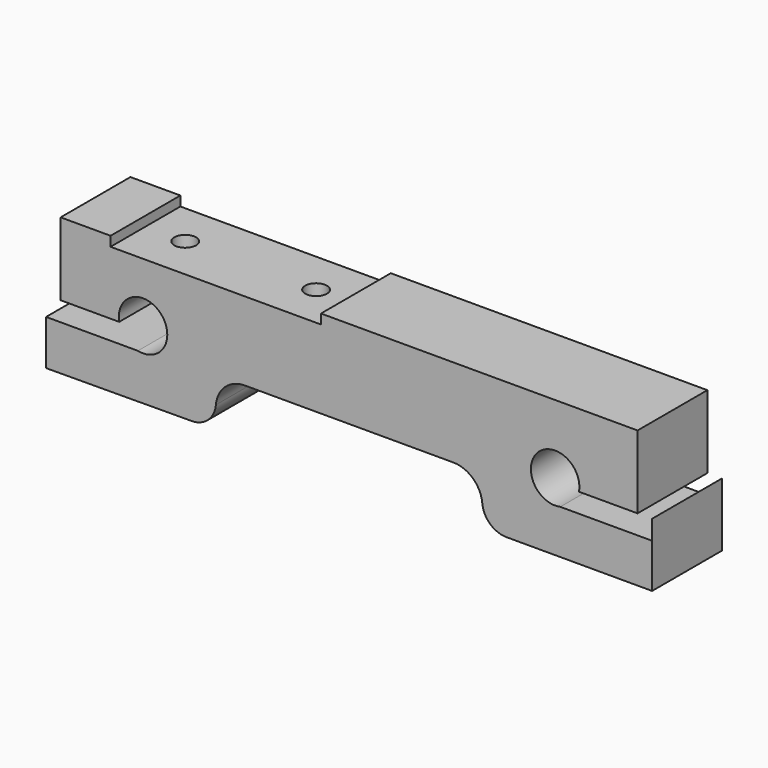
from build123d import *

# Parameters (mm, degrees)
F1_DEPTH = 18
F2_R     = 5
F3_R     = 2.25
F4_DEPTH = 8


# Not quite as in the source:
# - a feature names something its author has since deleted; it is built from what else it names


with BuildPart() as f1:
    # F0 (on Front) → F1 (new body)
    with BuildSketch(Plane.XZ):
        with BuildLine():
            ThreePointArc((-64.2237368111, 25.2650516673), (-59.7471801328, 31.1306109239), (-54.3027456241, 26.150402297))
            ThreePointArc((-54.3027456241, 26.150402297), (-56.1661028164, 22.2566288192), (-60.3673343828, 21.2650516673))
            Line((-60.3673343828, 21.2650516673), (-79.3032296173, 21.2650516673))
            Line((-79.3032296173, 21.2650516673), (-79.3043551346, 11.9631245031))
            Line((-79.3043551346, 11.9631245031), (-44.3043551346, 12.150402297))
            Line((-44.3043551346, 12.150402297), (-44.3043551346, 16.150402297))
            ThreePointArc((-44.3043551346, 16.150402297), (-42.5469958217, 20.3930429841), (-38.3043551346, 22.150402297))
            Line((-38.3043551346, 22.150402297), (4.6990865829, 22.150402297))
            ThreePointArc((4.6990865829, 22.150402297), (8.94172727, 20.3930429841), (10.6990865829, 16.150402297))
            Line((10.6990865829, 16.150402297), (10.6990865829, 12.150402297))
            Line((10.6990865829, 12.150402297), (45.6990865829, 12.150402297))
            Line((45.6990865829, 12.150402297), (45.6973702434, 25.2650516673))
            Line((45.6973702434, 25.2650516673), (45.6973702434, 21.2650516673))
            Line((45.6973702434, 21.2650516673), (42.6977375527, 21.2650516673))
            Line((42.6977375527, 21.2650516673), (26.7618431345, 21.2650516673))
            ThreePointArc((26.7618431345, 21.2650516673), (21.803480898, 29.2870451047), (30.6972543759, 26.150402297))
            ThreePointArc((30.6972543759, 26.150402297), (30.6774630028, 25.7059677883), (30.6182455629, 25.2650516673))
            Line((30.6182455629, 25.2650516673), (42.6977375527, 25.2650516673))
            Line((42.6977375527, 25.2650516673), (42.6977375527, 40.3215353384))
            Line((42.6977375527, 40.3215353384), (34.3958526514, 40.3215353384))
            Line((34.3958526514, 40.3215353384), (9.5622779218, 40.3215353384))
            Line((9.5622779218, 40.3215353384), (-22.6043551346, 40.3215353384))
            Line((-22.6043551346, 40.3215353384), (-22.6043551346, 38.3215353384))
            Line((-22.6043551346, 38.3215353384), (-44.3043551346, 38.3215353384))
            Line((-44.3043551346, 38.3215353384), (-66.0043551346, 38.3215353384))
            Line((-66.0043551346, 38.3215353384), (-66.0043551346, 40.3215353384))
            Line((-66.0043551346, 40.3215353384), (-76.3027456241, 40.3215353384))
            Line((-76.3027456241, 40.3215353384), (-76.3027456241, 25.2650516673))
            Line((-76.3027456241, 25.2650516673), (-64.2237368111, 25.2650516673))
        make_face()
    extrude(amount=F1_DEPTH)

    # F2
    f2_edges = [f1.edges().sort_by_distance(p)[0] for p in [
        (-44.304355, -9, 12.150402),
        (10.699087, -9, 12.150402),
    ]]
    fillet(f2_edges, radius=F2_R)

    # F3 (on face) → F4 (cut)
    with BuildSketch(Plane.XY.offset(38.3215353384)):
        with Locations((-30.8043551346, -9)):
            Circle(F3_R)
        with Locations((-57.8043551346, -9)):
            Circle(F3_R)
    extrude(amount=-F4_DEPTH, mode=Mode.SUBTRACT)


solid = f1.part
